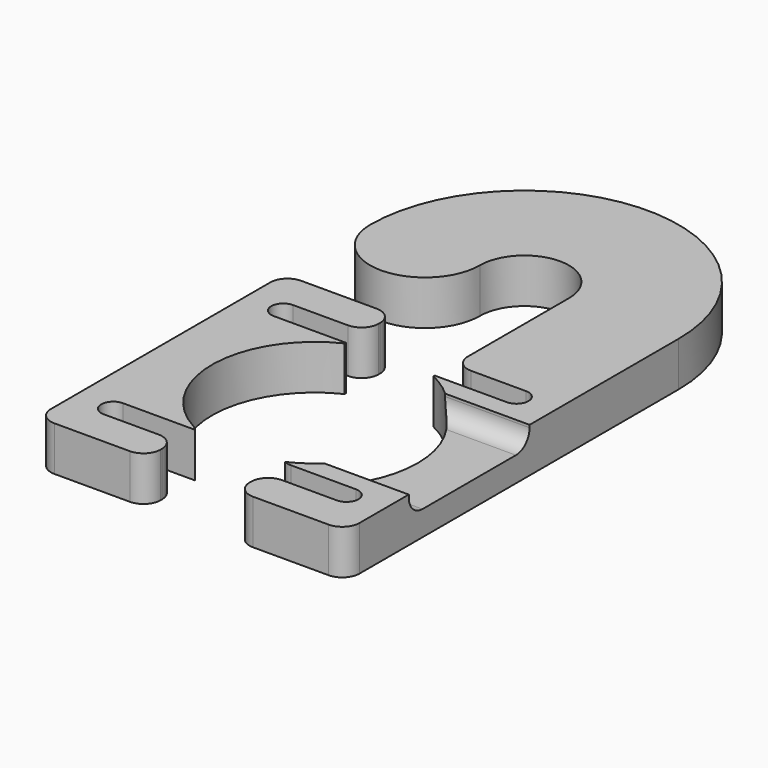
from build123d import *

# Parameters (mm, degrees)
F1_DEPTH       = 6.5
F2_W           = 22.0252647996
F2_H           = 8.9461854659
F3_DEPTH       = 33.6
F4_T1_DEPTH    = 19
F4_T3_DEPTH    = 10.5789393758
F4_2_T4_DEPTH  = 18.5656037181
F4_2_S5_R      = 15
F4_2_T6_DEPTH  = 11
F4_2_T10_DEPTH = 18.5656037181
F4_2_S11_R     = 15
F4_2_T12_DEPTH = 11
F4_2_T13_DEPTH = 19
F4_2_T15_DEPTH = 11.7124153355


# Not quite as in the source:
# - a fillet or chamfer that OpenCascade refuses, or shapes differently, is made with other operations: its cross-section is extruded or revolved along the edge and cut away or added


with BuildPart() as f1:
    # F0 (on Top) → F1 (new body)
    with BuildSketch(Plane.XY):
        with BuildLine():
            Line((-22.5, 22.5), (-22.5, -22.5))
            Line((-22.5, -22.5), (-6.4921572934, -22.5))
            Line((-6.4921572934, -22.5), (-6.4921572934, -17.25))
            Line((-6.4921572934, -17.25), (-17, -17.25))
            ThreePointArc((-17, -17.25), (-18.75, -15.5), (-17, -13.75))
            Line((-17, -13.75), (-6.4921572934, -13.75))
            Line((-6.4921572934, -13.75), (-6.4921572934, -13.5222739832))
            ThreePointArc((-6.4921572934, -13.5222739832), (-15, 0), (-6.4921572934, 13.5222739832))
            Line((-6.4921572934, 13.5222739832), (-6.4921572934, 13.75))
            Line((-6.4921572934, 13.75), (-17, 13.75))
            ThreePointArc((-17, 13.75), (-18.75, 15.5), (-17, 17.25))
            Line((-17, 17.25), (-6.4921572934, 17.25))
            Line((-6.4921572934, 17.25), (-6.4921572934, 22.5))
            Line((-6.4921572934, 22.5), (-22.5, 22.5))
        make_face()
    extrude(amount=F1_DEPTH)

    # F4: fillet of radius 2.5 on 11 edges, made by hand

    # F4_s2 → F4_t1 (cut)
    with BuildSketch(Plane.XY.offset(-6.25)):
        with BuildLine():
            ThreePointArc((-8.9921572934, -22.5), (-7.2243903405, -21.767766953), (-6.4921572934, -20))
            Line((-6.4921572934, -20), (-6.4421572934, -20))
            Line((-6.4421572934, -20), (-6.4421572934, -22.55))
            Line((-6.4421572934, -22.55), (-8.9921572934, -22.55))
            Line((-8.9921572934, -22.55), (-8.9921572934, -22.5))
        make_face()
        with BuildLine():
            ThreePointArc((-22.5, -20), (-21.767766953, -21.767766953), (-20, -22.5))
            Line((-20, -22.5), (-20, -22.55))
            Line((-20, -22.55), (-22.55, -22.55))
            Line((-22.55, -22.55), (-22.55, -20))
            Line((-22.55, -20), (-22.5, -20))
        make_face()
        with BuildLine():
            ThreePointArc((-8.9921572934, 17.25), (-7.2243903405, 17.982233047), (-6.4921572934, 19.75))
            Line((-6.4921572934, 19.75), (-6.4421572934, 19.75))
            Line((-6.4421572934, 19.75), (-6.4421572934, 17.2))
            Line((-6.4421572934, 17.2), (-8.9921572934, 17.2))
            Line((-8.9921572934, 17.2), (-8.9921572934, 17.25))
        make_face()
        with BuildLine():
            ThreePointArc((-6.4921572934, -19.75), (-7.2243903405, -17.982233047), (-8.9921572934, -17.25))
            Line((-8.9921572934, -17.25), (-8.9921572934, -17.2))
            Line((-8.9921572934, -17.2), (-6.4421572934, -17.2))
            Line((-6.4421572934, -17.2), (-6.4421572934, -19.75))
            Line((-6.4421572934, -19.75), (-6.4921572934, -19.75))
        make_face()
        with BuildLine():
            ThreePointArc((-20, 22.5), (-21.767766953, 21.767766953), (-22.5, 20))
            Line((-22.5, 20), (-22.55, 20))
            Line((-22.55, 20), (-22.55, 22.55))
            Line((-22.55, 22.55), (-20, 22.55))
            Line((-20, 22.55), (-20, 22.5))
        make_face()
        with BuildLine():
            ThreePointArc((-8.9921572934, 22.5), (-7.2243903405, 21.767766953), (-6.4921572934, 20))
            Line((-6.4921572934, 20), (-6.4421572934, 20))
            Line((-6.4421572934, 20), (-6.4421572934, 22.55))
            Line((-6.4421572934, 22.55), (-8.9921572934, 22.55))
            Line((-8.9921572934, 22.55), (-8.9921572934, 22.5))
        make_face()
    extrude(amount=F4_T1_DEPTH, mode=Mode.SUBTRACT)

    # F4_s4 → F4_t3 (cut)
    with BuildSketch(Plane.XY.offset(-2.0394696879)):
        with BuildLine():
            ThreePointArc((-6.4921572934, -13.75), (-6.8263856854, -13.4151830267), (-7.2177044937, -13.1493247675))
            Line((-7.2177044937, -13.1493247675), (-7.1936454787, -13.105493685))
            ThreePointArc((-7.1936454787, -13.105493685), (-6.8346085353, -13.2962636169), (-6.4705167691, -13.4771997366))
            Line((-6.4705167691, -13.4771997366), (-6.4421572934, -13.5222739832))
            ThreePointArc((-6.4421572934, -13.5222739832), (-6.4421572934, -13.6361369916), (-6.4535873345, -13.7181824221))
            Line((-6.4535873345, -13.7181824221), (-6.4921572934, -13.75))
        make_face()
    extrude(amount=F4_T3_DEPTH, mode=Mode.SUBTRACT)


with BuildPart() as f1b:
    # F0 (on Top) → F1, piece 2 (new body)
    with BuildSketch(Plane.XY):
        with BuildLine():
            Line((6.4921572934, -17.25), (6.4921572934, -22.5))
            Line((6.4921572934, -22.5), (22.5, -22.5))
            Line((22.5, -22.5), (22.5, 22.5))
            Line((22.5, 22.5), (6.4921572934, 22.5))
            Line((6.4921572934, 22.5), (6.4921572934, 17.25))
            Line((6.4921572934, 17.25), (17, 17.25))
            ThreePointArc((17, 17.25), (18.75, 15.5), (17, 13.75))
            Line((17, 13.75), (6.4921572934, 13.75))
            Line((6.4921572934, 13.75), (6.4921572934, 13.5222739832))
            ThreePointArc((6.4921572934, 13.5222739832), (12.6961088409, 7.9880423321), (15, 0))
            ThreePointArc((15, 0), (12.6961088409, -7.9880423321), (6.4921572934, -13.5222739832))
            Line((6.4921572934, -13.5222739832), (6.4921572934, -13.75))
            Line((6.4921572934, -13.75), (17, -13.75))
            ThreePointArc((17, -13.75), (18.75, -15.5), (17, -17.25))
            Line((17, -17.25), (6.4921572934, -17.25))
        make_face()
        with BuildLine():
            Line((6.4921572934, 38.1885590248), (6.4921572934, 22.5))
            Line((6.4921572934, 22.5), (22.5, 22.5))
            Line((22.5, 22.5), (22.5, 38.1885590248))
            ThreePointArc((22.5, 38.1885590248), (0, 60.6885590248), (-22.5, 38.1885590248))
            ThreePointArc((-22.5, 38.1885590248), (-14.4960786467, 30.1846376716), (-6.4921572934, 38.1885590248))
            ThreePointArc((-6.4921572934, 38.1885590248), (0, 44.6807163183), (6.4921572934, 38.1885590248))
        make_face()
    extrude(amount=F1_DEPTH)

    # F2 (on Right) → F3 (cut)
    with BuildSketch(Plane.YZ):
        with Locations((0, 8.0903784838)):
            Rectangle(F2_W, F2_H)
    extrude(amount=F3_DEPTH, mode=Mode.SUBTRACT)

    # F4#2: fillet of radius 2.5 on 11 edges, made by hand


with BuildPart() as f4_2_tool2:
    # F4_2_s3 → F4_2_t4 (new body)
    with BuildSketch(Plane.YZ.offset(3.9343962819)):
        with BuildLine():
            ThreePointArc((11.0126323998, 6.1172857508), (10.2803993528, 4.3495187978), (8.5126323998, 3.6172857508))
            Line((8.5126323998, 3.6172857508), (11.0126323998, 3.6172857508))
            Line((11.0126323998, 3.6172857508), (11.0126323998, 6.1172857508))
        make_face()
    extrude(amount=F4_2_T4_DEPTH)

    # F4_2_s5 → F4_2_t6 (cut, symmetric)
    with BuildSketch(Plane.XY.offset(4.9)):
        Circle(F4_2_S5_R)
    extrude(amount=F4_2_T6_DEPTH, both=True, mode=Mode.SUBTRACT)


with BuildPart() as f1b_1:
    add(f1b.part)

    # F4_2_t1: union F4_2_tool2
    add(f4_2_tool2.part)


with BuildPart() as f4_2_tool8:
    # F4_2_s9 → F4_2_t10 (new body)
    with BuildSketch(Plane.YZ.offset(3.9343962819)):
        with BuildLine():
            ThreePointArc((-11.0126323998, 6.1172857508), (-10.2803993528, 4.3495187978), (-8.5126323998, 3.6172857508))
            Line((-8.5126323998, 3.6172857508), (-11.0126323998, 3.6172857508))
            Line((-11.0126323998, 3.6172857508), (-11.0126323998, 6.1172857508))
        make_face()
    extrude(amount=F4_2_T10_DEPTH)

    # F4_2_s11 → F4_2_t12 (cut, symmetric)
    with BuildSketch(Plane.XY.offset(4.9)):
        Circle(F4_2_S11_R)
    extrude(amount=F4_2_T12_DEPTH, both=True, mode=Mode.SUBTRACT)


with BuildPart() as f1b_2:
    add(f1b_1.part)

    # F4_2_t7: union F4_2_tool8
    add(f4_2_tool8.part)

    # F4_2_s14 → F4_2_t13 (cut)
    with BuildSketch(Plane.XY.offset(-6.25)):
        with BuildLine():
            ThreePointArc((20, -22.5), (21.767766953, -21.767766953), (22.5, -20))
            Line((22.5, -20), (22.5, -22.5))
            Line((22.5, -22.5), (20, -22.5))
        make_face()
        with BuildLine():
            ThreePointArc((6.4921572934, -20), (7.2243903405, -21.767766953), (8.9921572934, -22.5))
            Line((8.9921572934, -22.5), (6.4921572934, -22.5))
            Line((6.4921572934, -22.5), (6.4921572934, -20))
        make_face()
        with BuildLine():
            ThreePointArc((6.4921572934, -19.75), (7.2243903405, -17.982233047), (8.9921572934, -17.25))
            Line((8.9921572934, -17.25), (6.4921572934, -17.25))
            Line((6.4921572934, -17.25), (6.4921572934, -19.75))
        make_face()
        with BuildLine():
            ThreePointArc((6.4921572934, 19.75), (7.2243903405, 17.982233047), (8.9921572934, 17.25))
            Line((8.9921572934, 17.25), (6.4921572934, 17.25))
            Line((6.4921572934, 17.25), (6.4921572934, 19.75))
        make_face()
    extrude(amount=F4_2_T13_DEPTH, mode=Mode.SUBTRACT)

    # F4_2_s16 → F4_2_t15 (cut)
    with BuildSketch(Plane.XY.offset(-2.6062076677)):
        with BuildLine():
            ThreePointArc((6.4921572934, -13.5222739832), (7.0011073054, -13.6924050604), (7.5346403605, -13.75))
            Line((7.5346403605, -13.75), (6.4921572934, -13.75))
            Line((6.4921572934, -13.75), (6.4921572934, -13.5222739832))
        make_face()
    extrude(amount=F4_2_T15_DEPTH, mode=Mode.SUBTRACT)


solid = Compound([f1.part, f1b_2.part])
